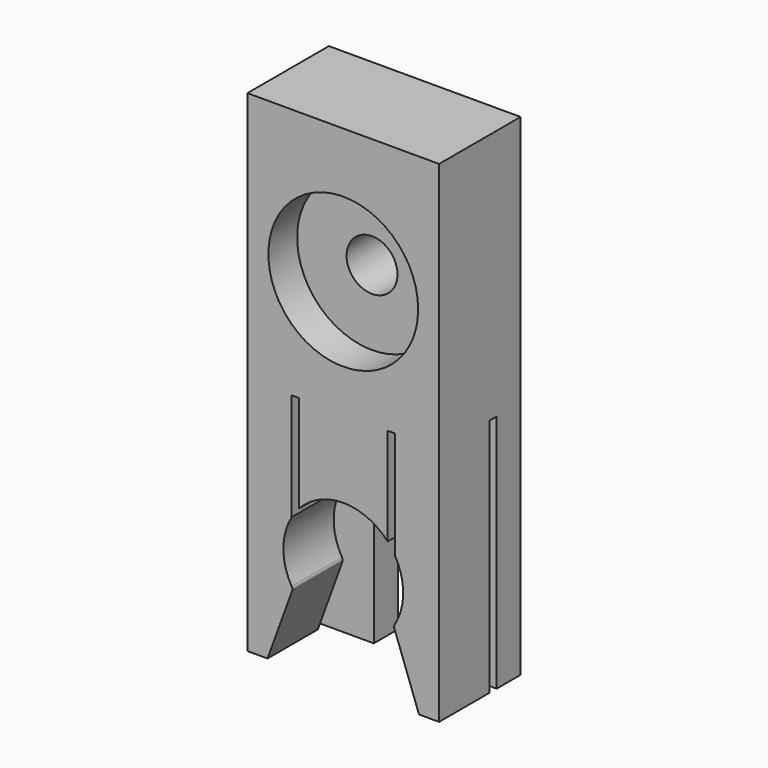
from build123d import *

# Parameters (mm, degrees)
F0_R     = 4.25
F1_DEPTH = 17
F2_DEPTH = 5
F4_DEPTH = 12
F5_W     = 4.6458135775
F5_H     = 1.5
F5_W_2   = 3.3541864225
F5_W_3   = 8
F6_DEPTH = 40
F7_R     = 12.5
F7_R_2   = 4.25
F8_DEPTH = 6


# Not quite as in the source:
# - a feature names something its author has since deleted; it is built from what else it names


with BuildPart() as f1:
    # F0 (on Front) → F1 (new body)
    with BuildSketch(Plane.XZ):
        with BuildLine():
            ThreePointArc((-8.5, -5.4772255751), (-8.5266357667, -5.2791241211), (-8.6046511628, -5.0950935582))
            ThreePointArc((-8.6046511628, -5.0950935582), (-9.9967746616, -5.5467065419), (-8.5452305344, -5.7337406825))
            ThreePointArc((-8.5452305344, -5.7337406825), (-8.5113941852, -5.6074617083), (-8.5, -5.4772255751))
        make_face()
        with BuildLine():
            ThreePointArc((-8.6046511628, -5.0950935582), (0, 10), (8.6046511628, -5.0950935582))
            ThreePointArc((8.6046511628, -5.0950935582), (9.4481014539, -4.7538613418), (10, -5.4772255751))
            ThreePointArc((10, -5.4772255751), (9.3802361333, -6.2158313898), (8.5452305344, -5.7337406825))
            Line((8.5452305344, -5.7337406825), (12.6458135775, -17))
            Line((12.6458135775, -17), (16, -17))
            Line((16, -17), (16, 65))
            Line((16, 65), (-16, 65))
            Line((-16, 65), (-16, -17))
            Line((-16, -17), (-12.6458135775, -17))
            Line((-12.6458135775, -17), (-8.5452305344, -5.7337406825))
            ThreePointArc((-8.5452305344, -5.7337406825), (-9.9967746616, -5.5467065419), (-8.6046511628, -5.0950935582))
        make_face()
        with Locations((0, 42.5)):
            Circle(F0_R, mode=Mode.SUBTRACT)
        with BuildLine():
            ThreePointArc((10, -5.4772255751), (9.4481014539, -4.7538613418), (8.6046511628, -5.0950935582))
            ThreePointArc((8.6046511628, -5.0950935582), (8.5032253384, -5.4077446082), (8.5452305344, -5.7337406825))
            ThreePointArc((8.5452305344, -5.7337406825), (9.3802361333, -6.2158313898), (10, -5.4772255751))
        make_face()
    extrude(amount=F1_DEPTH)

    # F0 (on Front) → F2 (join)
    with BuildSketch(Plane.XZ):
        with BuildLine():
            ThreePointArc((8.5452305344, -5.7337406825), (8.5032253384, -5.4077446082), (8.6046511628, -5.0950935582))
            ThreePointArc((8.6046511628, -5.0950935582), (0, 10), (-8.6046511628, -5.0950935582))
            ThreePointArc((-8.6046511628, -5.0950935582), (-8.5266357667, -5.2791241211), (-8.5, -5.4772255751))
            ThreePointArc((-8.5, -5.4772255751), (-8.5113941852, -5.6074617083), (-8.5452305344, -5.7337406825))
            Line((-8.5452305344, -5.7337406825), (-12.6458135775, -17))
            Line((-12.6458135775, -17), (-4.5, -17))
            Line((-4.5, -17), (-4.5, 0))
            ThreePointArc((-4.5, 0), (0, 4.5), (4.5, 0))
            Line((4.5, 0), (4.5, -17))
            Line((4.5, -17), (12.6458135775, -17))
            Line((12.6458135775, -17), (8.5452305344, -5.7337406825))
        make_face()
    extrude(amount=F2_DEPTH)

    # F3 (on face) → F4 (cut)
    with BuildSketch(Plane.XZ.offset(17)):
        with BuildLine():
            Line((-8.6046511628, 23), (-8.6046511628, 5.0950935582))
            ThreePointArc((-8.6046511628, 5.0950935582), (-8.0458244358, 5.938409648), (-7.4046511628, 6.7209479359))
            Line((-7.4046511628, 6.7209479359), (-7.4046511628, 23))
            Line((-7.4046511628, 23), (-8.6046511628, 23))
        make_face()
        with BuildLine():
            Line((7.4046511628, 23), (7.4046511628, 6.7209479359))
            ThreePointArc((7.4046511628, 6.7209479359), (8.0458244358, 5.938409648), (8.6046511628, 5.0950935582))
            Line((8.6046511628, 5.0950935582), (8.6046511628, 23))
            Line((8.6046511628, 23), (7.4046511628, 23))
        make_face()
    extrude(amount=-F4_DEPTH, mode=Mode.SUBTRACT)

    # F5 (on face) → F6 (cut)
    with BuildSketch(Plane(origin=(0, 0, -17), x_dir=(1, 0, 0), z_dir=(0, 0, -1))):
        with Locations((-10.3229067887, 5.75)):
            Rectangle(F5_W, F5_H)
        with Locations((-14.3229067887, 5.75)):
            Rectangle(F5_W_2, F5_H)
        with Locations((12, 5.75)):
            Rectangle(F5_W_3, F5_H)
    extrude(amount=-F6_DEPTH, mode=Mode.SUBTRACT)

    # F7 (on face) → F8 (cut)
    with BuildSketch(Plane.XZ.offset(17)):
        with Locations((0, 42.5)):
            Circle(F7_R)
        with Locations((0, 42.5)):
            Circle(F7_R_2, mode=Mode.SUBTRACT)
    extrude(amount=-F8_DEPTH, mode=Mode.SUBTRACT)


solid = f1.part
